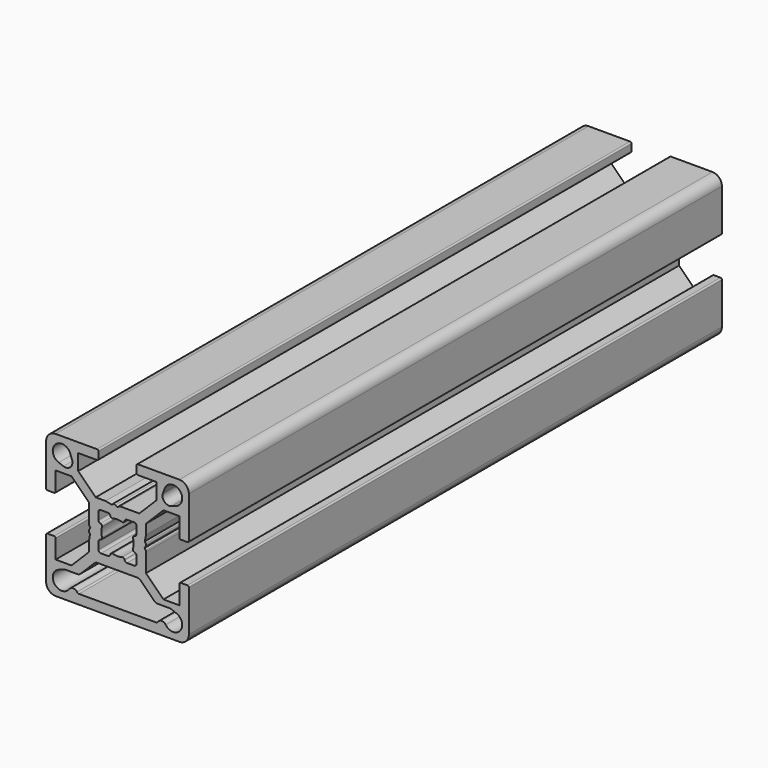
from build123d import *

# Parameters (mm, degrees)
F2_DEPTH = 70


# Not quite as in the source:
# - ends of sketch curves that miss each other by under 0.0002 mm in the source are joined


with BuildPart() as f2:
    # F1 (on Front) → F2 (new body, symmetric)
    with BuildSketch(Plane.XZ):
        with BuildLine():
            Line((8.249944, 9.6642), (4.58573, 5.999986))
            Line((4.58573, 5.999986), (0.653534, 5.999986))
            ThreePointArc((0.653534, 5.999986), (0.5241245494, 5.9829489324), (0.4035341291, 5.9329987764))
            Line((0.4035341291, 5.9329987764), (-5.6e-05, 5.699986))
            Line((-5.6e-05, 5.699986), (-0.403646, 5.932999))
            ThreePointArc((-0.403646, 5.932999), (-0.653646, 5.999986), (-0.9036458709, 5.9329987764))
            Line((-0.9036458709, 5.9329987764), (-1.218942, 5.750963))
            Line((-1.218942, 5.750963), (-2.500056, 5.999986))
            Line((-2.500056, 5.999986), (-4.585842, 5.999986))
            Line((-4.585842, 5.999986), (-8.250056, 9.6642))
            Line((-8.250056, 9.6642), (-8.250056, 12.999986))
            Line((-8.250056, 12.999986), (-4.300056, 12.999986))
            ThreePointArc((-4.300056, 12.999986), (-4.0879239656, 13.0878539656), (-4.000056, 13.299986))
            Line((-4.000056, 13.299986), (-4.000056, 14.699986))
            ThreePointArc((-4.000056, 14.699986), (-4.0879239656, 14.9121180344), (-4.300056, 14.999986))
            Line((-4.300056, 14.999986), (-13.000056, 14.999986))
            ThreePointArc((-13.000056, 14.999986), (-14.4142695624, 14.4141995624), (-15.000056, 12.999986))
            Line((-15.000056, 12.999986), (-15.000056, 4.299986))
            ThreePointArc((-15.000056, 4.299986), (-14.9121880344, 4.0878539656), (-14.700056, 3.999986))
            Line((-14.700056, 3.999986), (-13.300056, 3.999986))
            ThreePointArc((-13.300056, 3.999986), (-13.0879239656, 4.0878539656), (-13.000056, 4.299986))
            Line((-13.000056, 4.299986), (-13.000056, 8.249986))
            Line((-13.000056, 8.249986), (-9.66427, 8.249986))
            Line((-9.66427, 8.249986), (-6.000056, 4.585772))
            Line((-6.000056, 4.585772), (-6.000056, 0.653576))
            ThreePointArc((-6.000056, 0.653576), (-5.9830189324, 0.5241665494), (-5.9330687764, 0.4035761291))
            Line((-5.9330687764, 0.4035761291), (-5.700056, -1.4e-05))
            Line((-5.700056, -1.4e-05), (-5.933069, -0.403604))
            ThreePointArc((-5.933069, -0.403604), (-6.000056, -0.653604), (-5.9330687764, -0.9036038709))
            Line((-5.9330687764, -0.9036038709), (-5.751033, -1.2189))
            Line((-5.751033, -1.2189), (-6.000056, -2.500014))
            Line((-6.000056, -2.500014), (-6.000056, -4.5858))
            Line((-6.000056, -4.5858), (-9.66427, -8.250014))
            Line((-9.66427, -8.250014), (-13.000056, -8.250014))
            Line((-13.000056, -8.250014), (-13.000056, -4.300014))
            ThreePointArc((-13.000056, -4.300014), (-13.0879239656, -4.0878819656), (-13.300056, -4.000014))
            Line((-13.300056, -4.000014), (-14.700056, -4.000014))
            ThreePointArc((-14.700056, -4.000014), (-14.9121880344, -4.0878819656), (-15.000056, -4.300014))
            Line((-15.000056, -4.300014), (-15.000056, -13.000014))
            ThreePointArc((-15.000056, -13.000014), (-14.4142695624, -14.4142275624), (-13.000056, -15.000014))
            Line((-13.000056, -15.000014), (12.999944, -15.000014))
            ThreePointArc((12.999944, -15.000014), (14.4141575624, -14.4142275624), (14.999944, -13.000014))
            Line((14.999944, -13.000014), (14.999944, -4.300014))
            ThreePointArc((14.999944, -4.300014), (14.9120760344, -4.0878819656), (14.699944, -4.000014))
            Line((14.699944, -4.000014), (13.299944, -4.000014))
            ThreePointArc((13.299944, -4.000014), (13.0878119656, -4.0878819656), (12.999944, -4.300014))
            Line((12.999944, -4.300014), (12.999944, -8.250014))
            Line((12.999944, -8.250014), (9.664158, -8.250014))
            Line((9.664158, -8.250014), (5.999944, -4.5858))
            Line((5.999944, -4.5858), (5.999944, -0.653604))
            ThreePointArc((5.999944, -0.653604), (5.9829069324, -0.5241945494), (5.9329567764, -0.4036041291))
            Line((5.9329567764, -0.4036041291), (5.699944, -1.4e-05))
            Line((5.699944, -1.4e-05), (5.932957, 0.403576))
            ThreePointArc((5.932957, 0.403576), (5.999944, 0.653576), (5.9329567764, 0.9035758709))
            Line((5.9329567764, 0.9035758709), (5.750921, 1.218872))
            Line((5.750921, 1.218872), (5.999944, 2.499986))
            Line((5.999944, 2.499986), (5.999944, 4.585772))
            Line((5.999944, 4.585772), (9.664158, 8.249986))
            Line((9.664158, 8.249986), (12.999944, 8.249986))
            Line((12.999944, 8.249986), (12.999944, 4.299986))
            ThreePointArc((12.999944, 4.299986), (13.0878119656, 4.0878539656), (13.299944, 3.999986))
            Line((13.299944, 3.999986), (14.699944, 3.999986))
            ThreePointArc((14.699944, 3.999986), (14.9120760344, 4.0878539656), (14.999944, 4.299986))
            Line((14.999944, 4.299986), (14.999944, 12.999986))
            ThreePointArc((14.999944, 12.999986), (14.4141575624, 14.4141995624), (12.999944, 14.999986))
            Line((12.999944, 14.999986), (4.299944, 14.999986))
            ThreePointArc((4.299944, 14.999986), (4.0878119656, 14.9121180344), (3.999944, 14.699986))
            Line((3.999944, 14.699986), (3.999944, 13.299986))
            ThreePointArc((3.999944, 13.299986), (4.0878119656, 13.0878539656), (4.299944, 12.999986))
            Line((4.299944, 12.999986), (8.249944, 12.999986))
            Line((8.249944, 12.999986), (8.249944, 9.6642))
        make_face()
        with BuildLine():
            Line((-4.171629, -6.000014), (4.171517, -6.000014))
            ThreePointArc((4.171517, -6.000014), (4.5542004324, -6.0761344675), (4.8786237812, -6.2929072188))
            Line((4.8786237812, -6.2929072188), (7.742837, -9.157121))
            ThreePointArc((7.742837, -9.157121), (8.0672605676, -9.3738935325), (8.449944, -9.450014))
            Line((8.449944, -9.450014), (11.073348, -9.450014))
            Line((11.073348, -9.450014), (12.349782, -9.914598))
            ThreePointArc((12.349782, -9.914598), (13.2040603505, -12.8608903949), (10.1374570291, -12.7810479799))
            ThreePointArc((10.1374570291, -12.7810479799), (9.3136995047, -12.3500149751), (8.4911490608, -12.7833470418))
            ThreePointArc((8.4911490608, -12.7833470418), (8.3119125635, -12.9425444809), (8.079175, -13.000014))
            Line((8.079175, -13.000014), (-8.079287, -13.000014))
            ThreePointArc((-8.079287, -13.000014), (-8.3120245635, -12.9425444809), (-8.4912608636, -12.7833469062))
            ThreePointArc((-8.4912608636, -12.7833469062), (-9.3138115047, -12.3500149751), (-10.1375690315, -12.7810479782))
            ThreePointArc((-10.1375690315, -12.7810479782), (-13.2041723505, -12.8608903949), (-12.3498940253, -9.9145979306))
            Line((-12.3498940253, -9.9145979306), (-11.07346, -9.450014))
            Line((-11.07346, -9.450014), (-8.450056, -9.450014))
            ThreePointArc((-8.450056, -9.450014), (-8.0673725676, -9.3738935325), (-7.7429492188, -9.1571207812))
            Line((-7.7429492188, -9.1571207812), (-4.878736, -6.292907))
            ThreePointArc((-4.878736, -6.292907), (-4.5543124324, -6.0761344675), (-4.171629, -6.000014))
        make_face(mode=Mode.SUBTRACT)
        with BuildLine():
            ThreePointArc((-12.3498940253, 9.9145699306), (-13.0435588843, 13.0434888843), (-9.9146399306, 12.3498240253))
            Line((-9.9146399306, 12.3498240253), (-9.547908, 11.342236))
            ThreePointArc((-9.547908, 11.342236), (-9.8735275063, 9.8734575063), (-11.3423061215, 9.5478376661))
            Line((-11.3423061215, 9.5478376661), (-12.3498940253, 9.9145699306))
        make_face(mode=Mode.SUBTRACT)
        with BuildLine():
            ThreePointArc((0.9882629956, -3.2532009855), (-5.6e-05, -3.400014), (-0.9883749956, -3.2532009855))
            ThreePointArc((-0.9883749956, -3.2532009855), (-1.3178396431, -3.2974811593), (-1.5000564258, -3.5755229349))
            ThreePointArc((-1.5000564258, -3.5755229349), (-1.6685571025, -3.8793255231), (-1.994322, -4.000014))
            Line((-1.994322, -4.000014), (-3.500056, -4.000014))
            ThreePointArc((-3.500056, -4.000014), (-3.8536093906, -3.8535673906), (-4.000056, -3.500014))
            Line((-4.000056, -3.500014), (-4.000056, -1.99428))
            ThreePointArc((-4.000056, -1.99428), (-3.8793675231, -1.6685151025), (-3.5755649263, -1.5000144822))
            ThreePointArc((-3.5755649263, -1.5000144822), (-3.2975231593, -1.3177976431), (-3.2532441585, -0.9883290481))
            ThreePointArc((-3.2532441585, -0.9883290481), (-3.400056, -1.4e-05), (-3.2532429855, 0.9883049956))
            ThreePointArc((-3.2532429855, 0.9883049956), (-3.2975231593, 1.3177696431), (-3.5755649349, 1.4999864258))
            ThreePointArc((-3.5755649349, 1.4999864258), (-3.8793675231, 1.6684871025), (-4.000056, 1.994252))
            Line((-4.000056, 1.994252), (-4.000056, 3.499986))
            ThreePointArc((-4.000056, 3.499986), (-3.8536093906, 3.8535393906), (-3.500056, 3.999986))
            Line((-3.500056, 3.999986), (-1.994322, 3.999986))
            ThreePointArc((-1.994322, 3.999986), (-1.6685571025, 3.8792975231), (-1.5000564822, 3.5754949263))
            ThreePointArc((-1.5000564822, 3.5754949263), (-1.3178396431, 3.2974531593), (-0.9883710481, 3.2531741585))
            ThreePointArc((-0.9883710481, 3.2531741585), (-5.6e-05, 3.399986), (0.9882629956, 3.2531729855))
            ThreePointArc((0.9882629956, 3.2531729855), (1.3177276431, 3.2974531593), (1.4999444258, 3.5754949349))
            ThreePointArc((1.4999444258, 3.5754949349), (1.6684451025, 3.8792975231), (1.99421, 3.999986))
            Line((1.99421, 3.999986), (3.499944, 3.999986))
            ThreePointArc((3.499944, 3.999986), (3.8534973906, 3.8535393906), (3.999944, 3.499986))
            Line((3.999944, 3.499986), (3.999944, 1.994252))
            ThreePointArc((3.999944, 1.994252), (3.8792555231, 1.6684871025), (3.5754529263, 1.4999864822))
            ThreePointArc((3.5754529263, 1.4999864822), (3.2974111593, 1.3177696431), (3.2531321585, 0.9883010481))
            ThreePointArc((3.2531321585, 0.9883010481), (3.399944, -1.4e-05), (3.2531309855, -0.9883329956))
            ThreePointArc((3.2531309855, -0.9883329956), (3.2974111593, -1.3177976431), (3.5754529349, -1.5000144258))
            ThreePointArc((3.5754529349, -1.5000144258), (3.8792555231, -1.6685151025), (3.999944, -1.99428))
            Line((3.999944, -1.99428), (3.999944, -3.500014))
            ThreePointArc((3.999944, -3.500014), (3.8534973906, -3.8535673906), (3.499944, -4.000014))
            Line((3.499944, -4.000014), (1.99421, -4.000014))
            ThreePointArc((1.99421, -4.000014), (1.6684451025, -3.8793255231), (1.4999444822, -3.5755229263))
            ThreePointArc((1.4999444822, -3.5755229263), (1.3177276431, -3.2974811593), (0.9882629956, -3.2532009855))
        make_face(mode=Mode.SUBTRACT)
        with BuildLine():
            ThreePointArc((11.3421941215, 9.5478376661), (9.8734155063, 9.8734575063), (9.5477956661, 11.3422361215))
            Line((9.5477956661, 11.3422361215), (9.914528, 12.349824))
            ThreePointArc((9.914528, 12.349824), (13.0434468843, 13.0434888843), (12.3497820253, 9.9145699306))
            Line((12.3497820253, 9.9145699306), (11.3421941215, 9.5478376661))
        make_face(mode=Mode.SUBTRACT)
    extrude(amount=F2_DEPTH, both=True)


solid = f2.part
